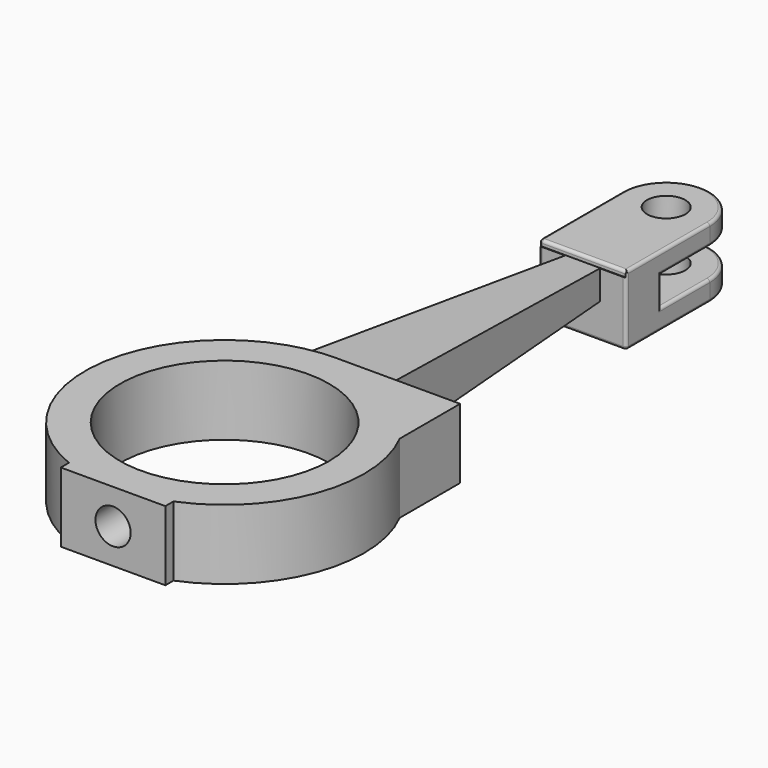
from build123d import *

# Parameters (mm, degrees)
F0_R           = 18
F1_DEPTH       = 12
F2_DEPTH       = 9.6
F0_R_2         = 3.3
F3_DEPTH       = 6
F3_DEPTH_BACK  = 6
F5_DEPTH       = 25
F5_DEPTH_BACK  = 25
F6_W           = 10.5
F6_H           = 5
F6_W_2         = 7.5
F7_DEPTH       = 25
F9_D           = 5
F9_DEPTH       = 17
F9_TIP         = 1.5021515476
F11_D          = 5
F11_DEPTH      = 17
F11_TIP        = 1.5021515476
F12_D          = 6.05
F12_DEPTH      = 17
F12_TIP        = 1.8176033726
F13_D          = 6.05
F13_DEPTH      = 17
F13_TIP        = 1.8176033726
F14_T1_DEPTH   = 5
F14_T3_DEPTH   = 10.5
F14_T5_DEPTH   = 17.5
F14_T7_DEPTH   = 11.7601440108
F14_T9_DEPTH   = 17.3832349181
F14_T11_DEPTH  = 14
F14_T13_DEPTH  = 19.1332349181
F14_T15_DEPTH  = 15.75
F14_S19_W      = 0.5
F14_S19_H      = 0.5
F14_T20_DEPTH  = 0.5
F14_S25_W      = 0.5
F14_S25_H      = 0.5
F14_T26_DEPTH  = 0.5
F14_S31_W      = 0.5
F14_S31_H      = 0.5
F14_T32_DEPTH  = 0.5
F14_T36_ANGLE  = 180
F14_T38_ANGLE  = 180
F14_T40_ANGLE  = 180
F14_T42_ANGLE  = 180
F14_T46_DEPTH  = 2.617204886
F14_T51_DEPTH  = 1.75
F14_T57_DEPTH  = 11.75
F14_T61_DEPTH  = 6.25
F14_T68_DEPTH  = 6.25
F14_T72_DEPTH  = 11.75
F14_T79_DEPTH  = 2.617204886
F14_T83_DEPTH  = 1.75
F14_T90_DEPTH  = 6.25
F14_T94_DEPTH  = 11.75
F14_T101_DEPTH = 11.75
F14_T105_DEPTH = 6.25


# Not quite as in the source:
# - a fillet or chamfer that OpenCascade refuses, or shapes differently, is made with other operations: its cross-section is extruded or revolved along the edge and cut away or added


with BuildPart() as f1:
    # F0 (on Top) → F1 (new body)
    with BuildSketch(Plane.XY):
        with BuildLine():
            Line((9, -24), (9, -22.2485954613))
            ThreePointArc((9, -22.2485954613), (22.5023455571, -8.3453247048), (21.3307290077, 11))
            Line((21.3307290077, 11), (21.3307290077, 24))
            Line((21.3307290077, 24), (7.4002087639, 24))
            Line((7.4002087639, 24), (0, 24))
            ThreePointArc((0, 24), (-3.7978527138, 23.6976014559), (-7.5, 22.7980262304))
            ThreePointArc((-7.5, 22.7980262304), (-23.9867053064, 0.7987293299), (-9, -22.2485954613))
            Line((-9, -22.2485954613), (-9, -24))
            Line((-9, -24), (9, -24))
        make_face()
        Circle(F0_R, mode=Mode.SUBTRACT)
    extrude(amount=F1_DEPTH)

    # F0 (on Top) → F2 (join)
    with BuildSketch(Plane.XY):
        with BuildLine():
            Line((0, 24), (7.4002087639, 24))
            Line((7.4002087639, 24), (3, 77))
            Line((3, 77), (-3, 77))
            Line((-3, 77), (-7.5, 22.7980262304))
            ThreePointArc((-7.5, 22.7980262304), (-3.7978527138, 23.6976014559), (0, 24))
        make_face()
    extrude(amount=F2_DEPTH)

    # F0 (on Top) → F3 (join, two sides)
    with BuildSketch(Plane.XY) as f3_sk:
        with BuildLine():
            Line((-3, 77), (3, 77))
            Line((3, 77), (7.5, 77))
            Line((7.5, 77), (7.5, 95))
            ThreePointArc((7.5, 95), (0, 102.5), (-7.5, 95))
            Line((-7.5, 95), (-7.5, 77))
            Line((-7.5, 77), (-3, 77))
        make_face()
        with Locations((0, 95)):
            Circle(F0_R_2, mode=Mode.SUBTRACT)
    extrude(amount=F3_DEPTH)
    extrude(f3_sk.sketch, amount=-F3_DEPTH_BACK)

    # F4 (on Right) → F5 (cut, two sides)
    with BuildSketch(Plane.YZ) as f5_sk:
        Polygon((24.0342058241, 9.6115674824), (77.1167650819, 5), (77.1167650819, 9.6115674824), align=None)
    extrude(amount=-F5_DEPTH, mode=Mode.SUBTRACT)
    extrude(f5_sk.sketch, amount=F5_DEPTH_BACK, mode=Mode.SUBTRACT)

    # F6 (on face) → F7 (cut)
    with BuildSketch(Plane.YZ.offset(7.5)):
        with Locations((89.75, 0)):
            Rectangle(F6_W, F6_H)
        with Locations((98.75, 0)):
            Rectangle(F6_W_2, F6_H)
    extrude(amount=-F7_DEPTH, mode=Mode.SUBTRACT)

    # F9
    with Locations(Plane.XZ.offset(24)):
        with Locations((0, 6)):
            Hole(F9_D / 2, depth=F9_DEPTH)
            with Locations((0, 0, -(F9_DEPTH + F9_TIP / 2))):  # 118° drill point
                Cone(0, F9_D / 2, F9_TIP, mode=Mode.SUBTRACT)

    # F11
    with Locations(Plane(origin=(0, 24, 0), x_dir=(-1, 0, 0), z_dir=(0, 1, 0))):
        with Locations((-15, 6)):
            Hole(F11_D / 2, depth=F11_DEPTH)
            with Locations((0, 0, -(F11_DEPTH + F11_TIP / 2))):  # 118° drill point
                Cone(0, F11_D / 2, F11_TIP, mode=Mode.SUBTRACT)

    # F12
    with Locations(Plane(origin=(0, 24, 0), x_dir=(-1, 0, 0), z_dir=(0, 1, 0))):
        with Locations((-15, 6)):
            Hole(F12_D / 2, depth=F12_DEPTH)
            with Locations((0, 0, -(F12_DEPTH + F12_TIP / 2))):  # 118° drill point
                Cone(0, F12_D / 2, F12_TIP, mode=Mode.SUBTRACT)

    # F13
    with Locations(Plane.XZ.offset(24)):
        with Locations((0, 6)):
            Hole(F13_D / 2, depth=F13_DEPTH)
            with Locations((0, 0, -(F13_DEPTH + F13_TIP / 2))):  # 118° drill point
                Cone(0, F13_D / 2, F13_TIP, mode=Mode.SUBTRACT)

    # F14: fillet of radius 0.5 on 22 edges, made by hand

    # F14_s2 → F14_t1 (cut)
    with BuildSketch(Plane.XY.offset(-2.5)):
        with BuildLine():
            ThreePointArc((-7.5, 84), (-7.3535533906, 84.3535533906), (-7, 84.5))
            Line((-7, 84.5), (-7.5, 84.5))
            Line((-7.5, 84.5), (-7.5, 84))
        make_face()
        with BuildLine():
            ThreePointArc((7.5, 84), (7.3535533906, 84.3535533906), (7, 84.5))
            Line((7, 84.5), (7.5, 84.5))
            Line((7.5, 84.5), (7.5, 84))
        make_face()
    extrude(amount=F14_T1_DEPTH, mode=Mode.SUBTRACT)

    # F14_s4 → F14_t3 (cut)
    with BuildSketch(Plane.XZ.offset(-95)):
        with BuildLine():
            ThreePointArc((-7.5, 3), (-7.3535533906, 2.6464466094), (-7, 2.5))
            Line((-7, 2.5), (-7.5, 2.5))
            Line((-7.5, 2.5), (-7.5, 3))
        make_face()
        with BuildLine():
            ThreePointArc((-7.5, -3), (-7.3535533906, -2.6464466094), (-7, -2.5))
            Line((-7, -2.5), (-7.5, -2.5))
            Line((-7.5, -2.5), (-7.5, -3))
        make_face()
        with BuildLine():
            ThreePointArc((7.5, -3), (7.3535533906, -2.6464466094), (7, -2.5))
            Line((7, -2.5), (7.5, -2.5))
            Line((7.5, -2.5), (7.5, -3))
        make_face()
        with BuildLine():
            ThreePointArc((7.5, 3), (7.3535533906, 2.6464466094), (7, 2.5))
            Line((7, 2.5), (7.5, 2.5))
            Line((7.5, 2.5), (7.5, 3))
        make_face()
    extrude(amount=F14_T3_DEPTH, mode=Mode.SUBTRACT)

    # F14_s6 → F14_t5 (cut)
    with BuildSketch(Plane.XZ.offset(-95)):
        with BuildLine():
            ThreePointArc((-7.5, -5.5), (-7.3535533906, -5.8535533906), (-7, -6))
            Line((-7, -6), (-7.5, -6))
            Line((-7.5, -6), (-7.5, -5.5))
        make_face()
        with BuildLine():
            ThreePointArc((7, -6), (7.3535533906, -5.8535533906), (7.5, -5.5))
            Line((7.5, -5.5), (7.5, -6))
            Line((7.5, -6), (7, -6))
        make_face()
    extrude(amount=F14_T5_DEPTH, mode=Mode.SUBTRACT)

    # F14_s8 → F14_t7 (cut)
    with BuildSketch(Plane.XY.offset(-5.5)):
        with BuildLine():
            ThreePointArc((-7, 77), (-7.3535533906, 77.1464466094), (-7.5, 77.5))
            Line((-7.5, 77.5), (-7.5, 77))
            Line((-7.5, 77), (-7, 77))
        make_face()
        with BuildLine():
            ThreePointArc((7, 77), (7.3535533906, 77.1464466094), (7.5, 77.5))
            Line((7.5, 77.5), (7.5, 77))
            Line((7.5, 77), (7, 77))
        make_face()
    extrude(amount=F14_T7_DEPTH, mode=Mode.SUBTRACT)

    # F14_s10 → F14_t9 (cut)
    with BuildSketch(Plane.XZ.offset(-95)):
        with BuildLine():
            ThreePointArc((-7.5, 5.5), (-7.3535533906, 5.8535533906), (-7, 6))
            Line((-7, 6), (-7.5, 6))
            Line((-7.5, 6), (-7.5, 5.5))
        make_face()
    extrude(amount=F14_T9_DEPTH, mode=Mode.SUBTRACT)

    # F14_s12 → F14_t11 (cut)
    with BuildSketch(Plane.YZ.offset(-7)):
        with BuildLine():
            ThreePointArc((77, -5.5), (77.1464466094, -5.8535533906), (77.5, -6))
            Line((77.5, -6), (77, -6))
            Line((77, -6), (77, -5.5))
        make_face()
    extrude(amount=F14_T11_DEPTH, mode=Mode.SUBTRACT)

    # F14_s14 → F14_t13 (cut)
    with BuildSketch(Plane.XZ.offset(-95)):
        with BuildLine():
            ThreePointArc((7.5, 5.5), (7.3535533906, 5.8535533906), (7, 6))
            Line((7, 6), (7.5, 6))
            Line((7.5, 6), (7.5, 5.5))
        make_face()
    extrude(amount=F14_T13_DEPTH, mode=Mode.SUBTRACT)

    # F14_s16 → F14_t15 (cut)
    with BuildSketch(Plane.YZ.offset(-7)):
        with BuildLine():
            ThreePointArc((77.1167650819, 5.5), (77.2632116913, 5.8535533906), (77.6167650819, 6))
            Line((77.6167650819, 6), (77.1167650819, 6))
            Line((77.1167650819, 6), (77.1167650819, 5.5))
        make_face()
    extrude(amount=F14_T15_DEPTH, mode=Mode.SUBTRACT)


with BuildPart() as f14_tool18:
    # F14_s19 → F14_t20 (new body)
    with BuildSketch(Plane.YZ.offset(-7)):
        with Locations((77.25, -5.75)):
            Rectangle(F14_S19_W, F14_S19_H)
    extrude(amount=-F14_T20_DEPTH)

    # F14_s21 → F14_t22 (revolve, cut)
    with BuildSketch(Plane(origin=(-7, 77.5, -5.5), x_dir=(0, 0.7071067812, 0.7071067812), z_dir=(0, -0.7071067812, 0.7071067812))):
        with BuildLine():
            ThreePointArc((0, -0.5), (0.5, 0), (0, 0.5))
            Line((0, 0.5), (0, -0.5))
        make_face()
    revolve(axis=Axis((-7, 77.5, -5.5), (-1, 0, 0)), mode=Mode.SUBTRACT)


with BuildPart() as f1_1:
    add(f1.part)

    # F14_t17: cut F14_tool18
    add(f14_tool18.part, mode=Mode.SUBTRACT)


with BuildPart() as f14_tool24:
    # F14_s25 → F14_t26 (new body)
    with BuildSketch(Plane.YZ.offset(-7)):
        with Locations((77.3667650819, 5.75)):
            Rectangle(F14_S25_W, F14_S25_H)
    extrude(amount=-F14_T26_DEPTH)

    # F14_s27 → F14_t28 (revolve, cut)
    with BuildSketch(Plane(origin=(-7, 77.6167650819, 5.5), x_dir=(0, 0.7071067812, -0.7071067812), z_dir=(0, 0.7071067812, 0.7071067812))):
        with BuildLine():
            ThreePointArc((0, -0.5), (0.5, 0), (0, 0.5))
            Line((0, 0.5), (0, -0.5))
        make_face()
    revolve(axis=Axis((-7, 77.6167650819, 5.5), (-1, 0, 0)), mode=Mode.SUBTRACT)


with BuildPart() as f1_2:
    add(f1_1.part)

    # F14_t23: cut F14_tool24
    add(f14_tool24.part, mode=Mode.SUBTRACT)


with BuildPart() as f14_tool30:
    # F14_s31 → F14_t32 (new body)
    with BuildSketch(Plane.YZ.offset(7)):
        with Locations((77.25, -5.75)):
            Rectangle(F14_S31_W, F14_S31_H)
    extrude(amount=F14_T32_DEPTH)

    # F14_s33 → F14_t34 (revolve, cut)
    with BuildSketch(Plane(origin=(7, 77.5, -5.5), x_dir=(0, 0.7071067812, 0.7071067812), z_dir=(0, 0.7071067812, -0.7071067812))):
        with BuildLine():
            ThreePointArc((0, -0.5), (0.5, 0), (0, 0.5))
            Line((0, 0.5), (0, -0.5))
        make_face()
    revolve(axis=Axis((7, 77.5, -5.5), (1, 0, 0)), mode=Mode.SUBTRACT)


with BuildPart() as f1_3:
    add(f1_2.part)

    # F14_t29: cut F14_tool30
    add(f14_tool30.part, mode=Mode.SUBTRACT)

    # F14_s35 → F14_t36 (revolve, cut)
    with BuildSketch(Plane.XZ.offset(-95)):
        with BuildLine():
            ThreePointArc((7, -2.5), (7.3535533906, -2.6464466094), (7.5, -3))
            Line((7.5, -3), (7.5, -2.5))
            Line((7.5, -2.5), (7, -2.5))
        make_face()
    revolve(axis=Axis((0, 95, -2.5), (0, 0, 1)), revolution_arc=F14_T36_ANGLE, mode=Mode.SUBTRACT)

    # F14_s37 → F14_t38 (revolve, cut)
    with BuildSketch(Plane.XZ.offset(-95)):
        with BuildLine():
            ThreePointArc((7.5, 3), (7.3535533906, 2.6464466094), (7, 2.5))
            Line((7, 2.5), (7.5, 2.5))
            Line((7.5, 2.5), (7.5, 3))
        make_face()
    revolve(axis=Axis((0, 95, 2.5), (0, 0, 1)), revolution_arc=F14_T38_ANGLE, mode=Mode.SUBTRACT)

    # F14_s39 → F14_t40 (revolve, cut)
    with BuildSketch(Plane.XZ.offset(-95)):
        with BuildLine():
            ThreePointArc((7.5, 5.5), (7.3535533906, 5.8535533906), (7, 6))
            Line((7, 6), (7.5, 6))
            Line((7.5, 6), (7.5, 5.5))
        make_face()
    revolve(axis=Axis((0, 95, 6), (0, 0, 1)), revolution_arc=F14_T40_ANGLE, mode=Mode.SUBTRACT)

    # F14_s41 → F14_t42 (revolve, cut)
    with BuildSketch(Plane.XZ.offset(-95)):
        with BuildLine():
            ThreePointArc((7, -6), (7.3535533906, -5.8535533906), (7.5, -5.5))
            Line((7.5, -5.5), (7.5, -6))
            Line((7.5, -6), (7, -6))
        make_face()
    revolve(axis=Axis((0, 95, -6), (0, 0, 1)), revolution_arc=F14_T42_ANGLE, mode=Mode.SUBTRACT)


with BuildPart() as f14_tool44:
    # F14_s45 → F14_t46 (new body)
    with BuildSketch(Plane(origin=(0, 74.74590152, -6.4935785634), x_dir=(1, 0, 0), z_dir=(0, 0.9962475616, -0.086549385))):
        with BuildLine():
            ThreePointArc((-7, -11.6556464009), (-7.3535533906, -11.5091997915), (-7.5, -11.1556464009))
            Line((-7.5, -11.1556464009), (-7.5, -11.6556464009))
            Line((-7.5, -11.6556464009), (-7, -11.6556464009))
        make_face()
    extrude(amount=F14_T46_DEPTH)

    split(bisect_by=Plane.XZ.offset(-77.1167650819), keep=Keep.TOP)


with BuildPart() as f1_4:
    add(f1_3.part)

    # F14_t43: cut F14_tool44
    add(f14_tool44.part, mode=Mode.SUBTRACT)


with BuildPart() as f14_tool49:
    # F14_s50 → F14_t51 (new body)
    with BuildSketch(Plane.XY.offset(3.75)):
        with BuildLine():
            ThreePointArc((-7.5, 77.6167650819), (-7.3535533906, 77.2632116913), (-7, 77.1167650819))
            Line((-7, 77.1167650819), (-7.5, 77.1167650819))
            Line((-7.5, 77.1167650819), (-7.5, 77.6167650819))
        make_face()
    extrude(amount=F14_T51_DEPTH)

    split(bisect_by=Plane(origin=(0, 1.0087890281, 11.6119093055), x_dir=(1, 0, 0), z_dir=(0, 0.086549385, 0.9962475616)), keep=Keep.TOP)


with BuildPart() as f1_5:
    add(f1_4.part)

    # F14_t48: cut F14_tool49
    add(f14_tool49.part, mode=Mode.SUBTRACT)


with BuildPart() as f14_tool55:
    # F14_s56 → F14_t57 (new body)
    with BuildSketch(Plane.XZ.offset(-95)):
        with BuildLine():
            ThreePointArc((-7.5, 3), (-7.3535533906, 2.6464466094), (-7, 2.5))
            Line((-7, 2.5), (-7.5, 2.5))
            Line((-7.5, 2.5), (-7.5, 3))
        make_face()
    extrude(amount=F14_T57_DEPTH)

    split(bisect_by=Plane.XZ.offset(-84.5), keep=Keep.TOP)


with BuildPart() as f14_tool59:
    # F14_s60 → F14_t61 (new body)
    with BuildSketch(Plane.XY.offset(3.75)):
        with BuildLine():
            ThreePointArc((-7.5, 84), (-7.3535533906, 84.3535533906), (-7, 84.5))
            Line((-7, 84.5), (-7.5, 84.5))
            Line((-7.5, 84.5), (-7.5, 84))
        make_face()
    extrude(amount=-F14_T61_DEPTH)

    split(bisect_by=Plane.XY.offset(2.5), keep=Keep.TOP)


with BuildPart() as f14_tool55_1:
    add(f14_tool55.part)

    # F14_t63: intersect F14_tool59
    add(f14_tool59.part, mode=Mode.INTERSECT)


with BuildPart() as f1_6:
    add(f1_5.part)

    # F14_t53: cut F14_tool55
    add(f14_tool55_1.part, mode=Mode.SUBTRACT)


with BuildPart() as f14_tool66:
    # F14_s67 → F14_t68 (new body)
    with BuildSketch(Plane.XY.offset(2.5)):
        with BuildLine():
            ThreePointArc((-7.5, 84), (-7.3535533906, 84.3535533906), (-7, 84.5))
            Line((-7, 84.5), (-7.5, 84.5))
            Line((-7.5, 84.5), (-7.5, 84))
        make_face()
    extrude(amount=-F14_T68_DEPTH)

    split(bisect_by=Plane.XY.offset(-2.5), keep=Keep.BOTTOM)


with BuildPart() as f14_tool70:
    # F14_s71 → F14_t72 (new body)
    with BuildSketch(Plane.XZ.offset(-83.25)):
        with BuildLine():
            ThreePointArc((-7.5, -3), (-7.3535533906, -2.6464466094), (-7, -2.5))
            Line((-7, -2.5), (-7.5, -2.5))
            Line((-7.5, -2.5), (-7.5, -3))
        make_face()
    extrude(amount=-F14_T72_DEPTH)

    split(bisect_by=Plane.XZ.offset(-84.5), keep=Keep.TOP)


with BuildPart() as f14_tool66_1:
    add(f14_tool66.part)

    # F14_t74: intersect F14_tool70
    add(f14_tool70.part, mode=Mode.INTERSECT)


with BuildPart() as f1_7:
    add(f1_6.part)

    # F14_t64: cut F14_tool66
    add(f14_tool66_1.part, mode=Mode.SUBTRACT)


with BuildPart() as f14_tool77:
    # F14_s78 → F14_t79 (new body)
    with BuildSketch(Plane(origin=(0, 74.74590152, -6.4935785634), x_dir=(1, 0, 0), z_dir=(0, 0.9962475616, -0.086549385))):
        with BuildLine():
            ThreePointArc((-7, -11.6556464009), (-7.3535533906, -11.5091997915), (-7.5, -11.1556464009))
            Line((-7.5, -11.1556464009), (-7.5, -11.6556464009))
            Line((-7.5, -11.6556464009), (-7, -11.6556464009))
        make_face()
    extrude(amount=F14_T79_DEPTH)

    split(bisect_by=Plane.XZ.offset(-77.1167650819), keep=Keep.BOTTOM)


with BuildPart() as f14_tool81:
    # F14_s82 → F14_t83 (new body)
    with BuildSketch(Plane.XY.offset(3.75)):
        with BuildLine():
            ThreePointArc((-7.5, 77.6167650819), (-7.3535533906, 77.2632116913), (-7, 77.1167650819))
            Line((-7, 77.1167650819), (-7.5, 77.1167650819))
            Line((-7.5, 77.1167650819), (-7.5, 77.6167650819))
        make_face()
    extrude(amount=F14_T83_DEPTH)

    split(bisect_by=Plane(origin=(0, 1.0087890281, 11.6119093055), x_dir=(1, 0, 0), z_dir=(0, -0.086549385, -0.9962475616)), keep=Keep.TOP)


with BuildPart() as f14_tool77_1:
    add(f14_tool77.part)

    # F14_t85: intersect F14_tool81
    add(f14_tool81.part, mode=Mode.INTERSECT)


with BuildPart() as f1_8:
    add(f1_7.part)

    # F14_t75: cut F14_tool77
    add(f14_tool77_1.part, mode=Mode.SUBTRACT)


with BuildPart() as f14_tool88:
    # F14_s89 → F14_t90 (new body)
    with BuildSketch(Plane.XY.offset(3.75)):
        with BuildLine():
            ThreePointArc((7.5, 84), (7.3535533906, 84.3535533906), (7, 84.5))
            Line((7, 84.5), (7.5, 84.5))
            Line((7.5, 84.5), (7.5, 84))
        make_face()
    extrude(amount=-F14_T90_DEPTH)

    split(bisect_by=Plane.XY.offset(2.5), keep=Keep.TOP)


with BuildPart() as f14_tool92:
    # F14_s93 → F14_t94 (new body)
    with BuildSketch(Plane.XZ.offset(-95)):
        with BuildLine():
            ThreePointArc((7.5, 3), (7.3535533906, 2.6464466094), (7, 2.5))
            Line((7, 2.5), (7.5, 2.5))
            Line((7.5, 2.5), (7.5, 3))
        make_face()
    extrude(amount=F14_T94_DEPTH)

    split(bisect_by=Plane.XZ.offset(-84.5), keep=Keep.TOP)


with BuildPart() as f14_tool88_1:
    add(f14_tool88.part)

    # F14_t96: intersect F14_tool92
    add(f14_tool92.part, mode=Mode.INTERSECT)


with BuildPart() as f1_9:
    add(f1_8.part)

    # F14_t86: cut F14_tool88
    add(f14_tool88_1.part, mode=Mode.SUBTRACT)


with BuildPart() as f14_tool99:
    # F14_s100 → F14_t101 (new body)
    with BuildSketch(Plane.XZ.offset(-83.25)):
        with BuildLine():
            ThreePointArc((7.5, -3), (7.3535533906, -2.6464466094), (7, -2.5))
            Line((7, -2.5), (7.5, -2.5))
            Line((7.5, -2.5), (7.5, -3))
        make_face()
    extrude(amount=-F14_T101_DEPTH)

    split(bisect_by=Plane.XZ.offset(-84.5), keep=Keep.TOP)


with BuildPart() as f14_tool103:
    # F14_s104 → F14_t105 (new body)
    with BuildSketch(Plane.XY.offset(2.5)):
        with BuildLine():
            ThreePointArc((7.5, 84), (7.3535533906, 84.3535533906), (7, 84.5))
            Line((7, 84.5), (7.5, 84.5))
            Line((7.5, 84.5), (7.5, 84))
        make_face()
    extrude(amount=-F14_T105_DEPTH)

    split(bisect_by=Plane.XY.offset(-2.5), keep=Keep.BOTTOM)


with BuildPart() as f14_tool99_1:
    add(f14_tool99.part)

    # F14_t107: intersect F14_tool103
    add(f14_tool103.part, mode=Mode.INTERSECT)


with BuildPart() as f1_10:
    add(f1_9.part)

    # F14_t97: cut F14_tool99
    add(f14_tool99_1.part, mode=Mode.SUBTRACT)


solid = f1_10.part
